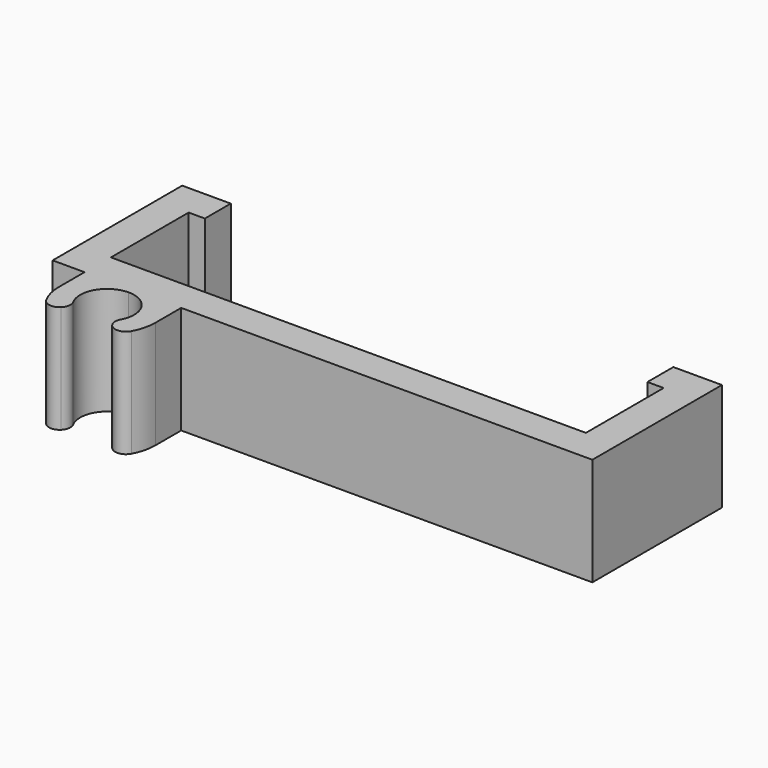
from build123d import *

# Parameters (mm, degrees)
F1_DEPTH    = 10
F2_T1_DEPTH = 16.5073043021
F2_T3_DEPTH = 14.2705098312


# Not quite as in the source:
# - a fillet or chamfer that OpenCascade refuses, or shapes differently, is made with other operations: its cross-section is extruded or revolved along the edge and cut away or added


with BuildPart() as f1:
    # F0 (on Top) → F1 (new body)
    with BuildSketch(Plane.XY):
        with BuildLine():
            Line((-25.6786430255, 0), (12.4131741374, 0))
            Line((12.4131741374, 0), (12.4131741374, 15))
            Line((12.4131741374, 15), (7.9131741374, 15))
            Line((7.9131741374, 15), (7.9131741374, 12))
            Line((7.9131741374, 12), (9.4131741374, 12))
            Line((9.4131741374, 12), (9.4131741374, 3))
            Line((9.4131741374, 3), (-34.5868258626, 3))
            Line((-34.5868258626, 3), (-34.5868258626, 12))
            Line((-34.5868258626, 12), (-33.0868258626, 12))
            Line((-33.0868258626, 12), (-33.0868258626, 15))
            Line((-33.0868258626, 15), (-37.5868258626, 15))
            Line((-37.5868258626, 15), (-37.5868258626, 0))
            Line((-37.5868258626, 0), (-34.6318436787, 0))
            Line((-34.6318436787, 0), (-34.6318436787, -2.9766003136))
            ThreePointArc((-34.6318436787, -2.9766003136), (-34.291082769, -4.6897210919), (-33.3206777997, -6.1420347612))
            Line((-33.3206777997, -6.1420347612), (-31.923010305, -4.7443672665))
            ThreePointArc((-31.923010305, -4.7443672665), (-32.4649421833, -2.0198917326), (-30.1552433521, -0.4766003136))
            ThreePointArc((-30.1552433521, -0.4766003136), (-27.8455445208, -2.0198917326), (-28.3874763991, -4.7443672665))
            Line((-28.3874763991, -4.7443672665), (-26.9898089045, -6.1420347612))
            ThreePointArc((-26.9898089045, -6.1420347612), (-26.0194039351, -4.6897210919), (-25.6786430255, -2.9766003136))
            Line((-25.6786430255, -2.9766003136), (-25.6786430255, 0))
        make_face()
    extrude(amount=F1_DEPTH)

    # F2: fillet of radius 1 on 4 edges, made by hand

    # F2_s2 → F2_t1 (cut)
    with BuildSketch(Plane.XY.offset(-3.253652151)):
        with BuildLine():
            ThreePointArc((-32.5096806342, -5.3310375957), (-33.3621500528, -5.6133092576), (-34.0974017442, -5.0977645446))
            ThreePointArc((-34.0974017442, -5.0977645446), (-33.7471918574, -5.6482770191), (-33.3206777997, -6.1420347612))
            Line((-33.3206777997, -6.1420347612), (-32.5096806342, -5.3310375957))
        make_face()
        with BuildLine():
            ThreePointArc((-27.8008060699, -5.3310375957), (-26.9483366513, -5.6133092576), (-26.2130849599, -5.0977645446))
            ThreePointArc((-26.2130849599, -5.0977645446), (-26.5632948467, -5.6482770191), (-26.9898089045, -6.1420347612))
            Line((-26.9898089045, -6.1420347612), (-27.8008060699, -5.3310375957))
        make_face()
    extrude(amount=F2_T1_DEPTH, mode=Mode.SUBTRACT)

    # F2_s4 → F2_t3 (cut)
    with BuildSketch(Plane.XY.offset(-2.1352549156)):
        with BuildLine():
            ThreePointArc((-32.5269515972, -5.3483085587), (-32.2445345415, -4.7855713596), (-32.3543969423, -4.1656013592))
            ThreePointArc((-32.3543969423, -4.1656013592), (-32.1597026664, -4.4706360752), (-31.923010305, -4.7443672665))
            Line((-31.923010305, -4.7443672665), (-32.5269515972, -5.3483085587))
        make_face()
        with BuildLine():
            ThreePointArc((-27.9560897618, -4.1656013592), (-28.0659521626, -4.7855713596), (-27.7835351069, -5.3483085587))
            Line((-27.7835351069, -5.3483085587), (-28.3874763991, -4.7443672665))
            ThreePointArc((-28.3874763991, -4.7443672665), (-28.1507840377, -4.4706360752), (-27.9560897618, -4.1656013592))
        make_face()
    extrude(amount=F2_T3_DEPTH, mode=Mode.SUBTRACT)


solid = f1.part
